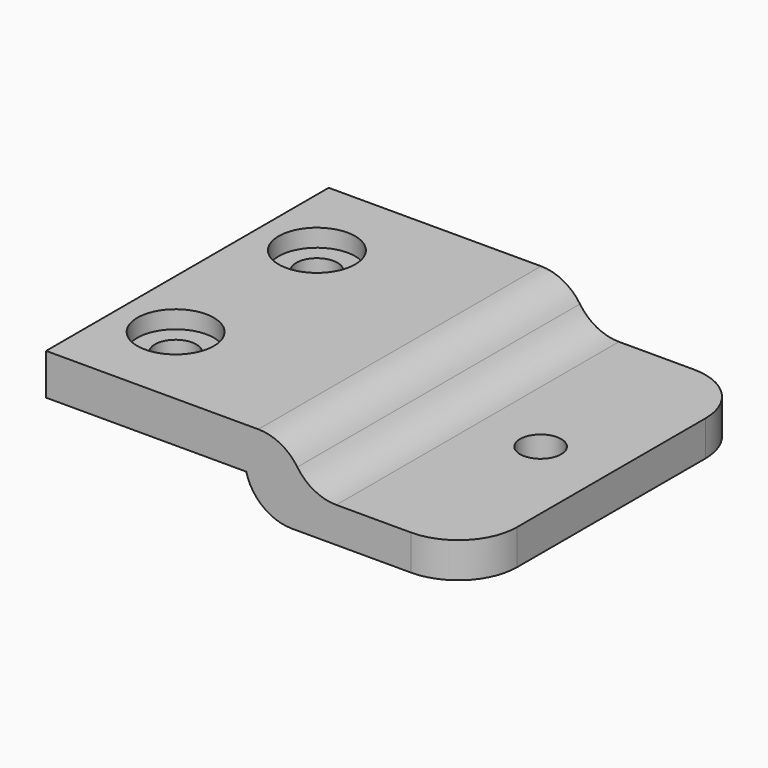
from build123d import *

# Parameters (mm, degrees)
F0_W        = 5
F0_H        = 30
F0_W_2      = 17
F0_R        = 1.75
F1_DEPTH    = 3.5
F2_DEPTH    = 3
F3_T1_DEPTH = 49.843134833
F3_T3_DEPTH = 49.364916731
F4_R        = 3.25
F5_DEPTH    = 1.5
F6_R        = 4


# Not quite as in the source:
# - a fillet or chamfer that OpenCascade refuses, or shapes differently, is made with other operations: its cross-section is extruded or revolved along the edge and cut away or added


with BuildPart() as f1:
    # F0 (on Top) → F1 (new body)
    with BuildSketch(Plane.XY):
        Rectangle(F0_W, F0_H)
        with Locations((-11, 0)):
            Rectangle(F0_W_2, F0_H)
        with Locations((-14.5, -7.5)):
            Circle(F0_R, mode=Mode.SUBTRACT)
        with Locations((-14.5, 7.5)):
            Circle(F0_R, mode=Mode.SUBTRACT)
    extrude(amount=F1_DEPTH)

    # F0 (on Top) → F2 (join)
    with BuildSketch(Plane.XY):
        with BuildLine():
            Line((11.5, 15), (2.5, 15))
            Line((2.5, 15), (2.5, -15))
            Line((2.5, -15), (11.5, -15))
            ThreePointArc((11.5, -15), (15.0355339059, -13.5355339059), (16.5, -10))
            Line((16.5, -10), (16.5, 10))
            ThreePointArc((16.5, 10), (15.0355339059, 13.5355339059), (11.5, 15))
        make_face()
        with Locations((10.5, 0)):
            Circle(F0_R, mode=Mode.SUBTRACT)
        Rectangle(F0_W, F0_H)
    extrude(amount=-F2_DEPTH)

    # F3: fillet of radius 4 on 2 edges, made by hand

    # F3_s2 → F3_t1 (cut)
    with BuildSketch(Plane.XZ.offset(-24.9215674165)):
        with BuildLine():
            ThreePointArc((2.5, 0), (1.1771243445, 2.5), (-1.4686269666, 3.5))
            Line((-1.4686269666, 3.5), (2.5, 3.5))
            Line((2.5, 3.5), (2.5, 0))
        make_face()
    extrude(amount=F3_T1_DEPTH, mode=Mode.SUBTRACT)

    # F3_s4 → F3_t3 (cut)
    with BuildSketch(Plane.XZ.offset(-24.6824583655)):
        with BuildLine():
            ThreePointArc((-2.5, 0), (-1.0765063966, -2.1622776602), (1.3729833462, -3))
            Line((1.3729833462, -3), (-2.5, -3))
            Line((-2.5, -3), (-2.5, 0))
        make_face()
    extrude(amount=F3_T3_DEPTH, mode=Mode.SUBTRACT)

    # F4 (on face) → F5 (cut)
    with BuildSketch(Plane.XY.offset(3.5)):
        with Locations((-14.5, 7.5)):
            Circle(F4_R)
        with Locations((-14.5, -7.5)):
            Circle(F4_R)
    extrude(amount=-F5_DEPTH, mode=Mode.SUBTRACT)

    # F6
    f6_edges = [f1.edges().sort_by_distance(p)[0] for p in [
        (2.5, 0, 0),
    ]]
    fillet(f6_edges, radius=F6_R)


solid = f1.part
